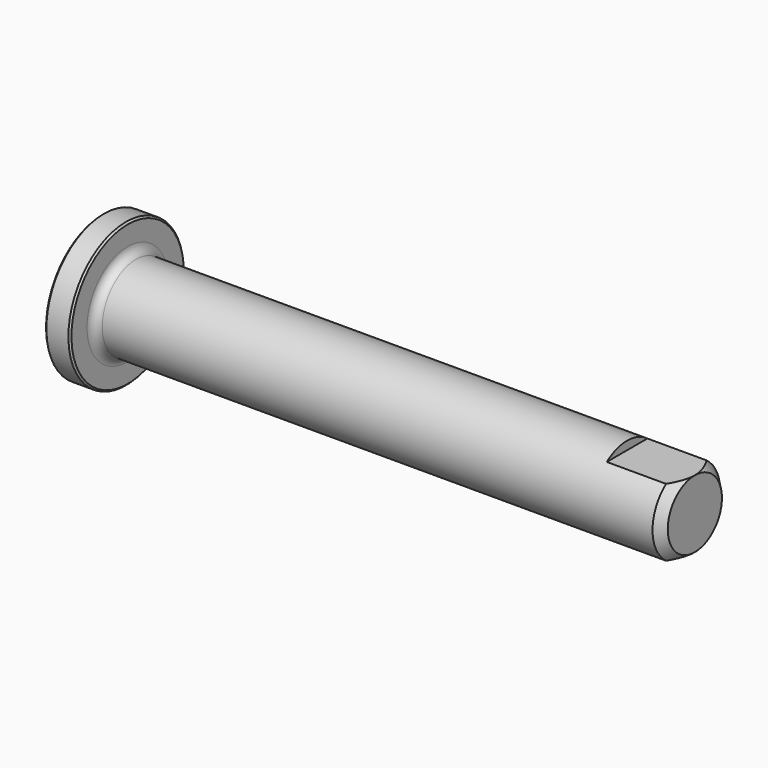
from build123d import *

# Parameters (mm, degrees)
F2_SIZE  = 0.2
F3_SIZE  = 1
F4_R     = 1
F5_W     = 8
F5_H     = 1
F6_DEPTH = 12.5


# Not quite as in the source:
# - a pattern or mirror of a feature is missing from the dataset's text; its kind, count and spacing are read off the source's solid


with BuildPart() as f1:
    # F0 (on Front) → F1 (revolve)
    with BuildSketch(Plane.XZ):
        Polygon((-3, 8.5), (-3, 0), (67, 0), (67, 5), (0, 5), (0, 8.5), align=None)
    revolve(axis=Axis((32, 0, 0), (-1, 0, 0)))

    # F2
    f2_edges = [f1.edges().sort_by_distance(p)[0] for p in [
        (0, 0, -8.5),
        (-3, 0, -8.5),
    ]]
    chamfer(f2_edges, length=F2_SIZE)

    # F3
    f3_edges = [f1.edges().sort_by_distance(p)[0] for p in [
        (67, 0, -5),
    ]]
    chamfer(f3_edges, length=F3_SIZE)

    # F4
    f4_edges = [f1.edges().sort_by_distance(p)[0] for p in [
        (0, 0, -5),
    ]]
    fillet(f4_edges, radius=F4_R)

    # F5 (on Front) → F6 (cut, symmetric)
    with BuildSketch(Plane.XZ):
        with Locations((63, 4.5)):
            Rectangle(F5_W, F5_H)
    f6 = extrude(amount=F6_DEPTH, both=True, mode=Mode.SUBTRACT)

    # F6_copies: F6 across plane
    add(f6.mirror(Plane(origin=(0, 0, 0), x_dir=(-1, 0, 0), z_dir=(0, 0, -1))), mode=Mode.SUBTRACT)


solid = f1.part
